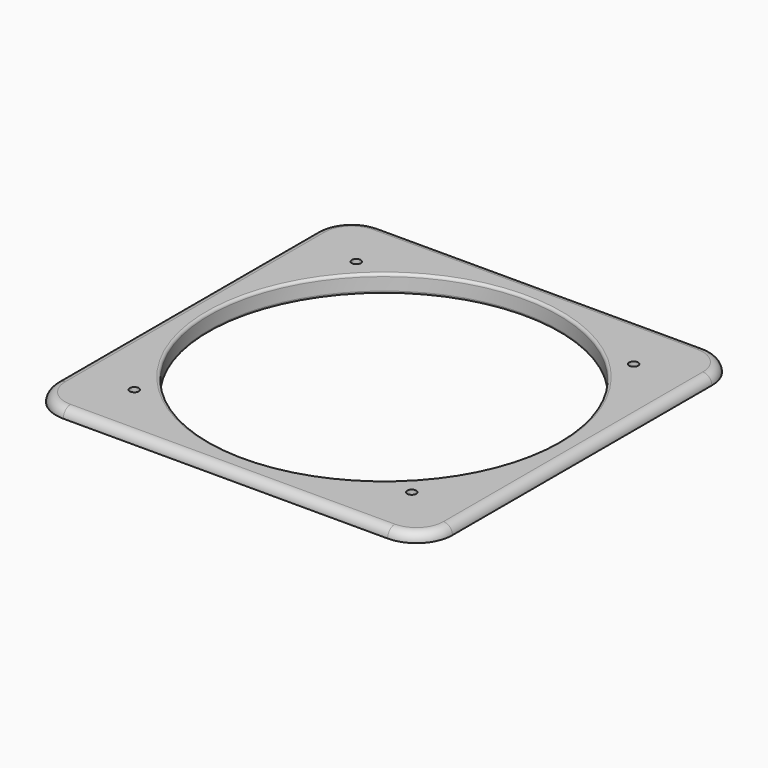
from build123d import *

# Parameters (mm, degrees)
F0_R     = 97
F1_DEPTH = 5
F3_R     = 102
F3_R_2   = 97
F4_DEPTH = 5
F5_R     = 1.5
F6_R     = 4.99999
F2_R     = 2.5
F7_DEPTH = 5


# Not quite as in the source:
# - a fillet or chamfer is up to 0.001 mm smaller than in the source, because OpenCascade refuses the exact size


with BuildPart() as f1:
    # F0 (on Top) → F1 (new body)
    with BuildSketch(Plane.XY):
        with BuildLine():
            Line((-90, -110), (90, -110))
            ThreePointArc((90, -110), (104.1421356237, -104.1421356237), (110, -90))
            Line((110, -90), (110, 90))
            ThreePointArc((110, 90), (104.1421356237, 104.1421356237), (90, 110))
            Line((90, 110), (-90, 110))
            ThreePointArc((-90, 110), (-104.1421356237, 104.1421356237), (-110, 90))
            Line((-110, 90), (-110, -90))
            ThreePointArc((-110, -90), (-104.1421356237, -104.1421356237), (-90, -110))
        make_face()
        Circle(F0_R, mode=Mode.SUBTRACT)
    extrude(amount=F1_DEPTH)

    # F3 (on face) → F4 (join)
    with BuildSketch(Plane(origin=(0, 0, 0), x_dir=(1, 0, 0), z_dir=(0, 0, -1))):
        Circle(F3_R)
        Circle(F3_R_2, mode=Mode.SUBTRACT)
    extrude(amount=F4_DEPTH)

    # F5
    f5_edges = [f1.edges().sort_by_distance(p)[0] for p in [
        (-97, 0, -5),
        (-102, 0, -5),
        (-97, 0, 5),
    ]]
    fillet(f5_edges, radius=F5_R)

    # F6 (radius 5 in the source; OpenCascade refuses exactly that, so slightly less here)
    f6_edges = [f1.edges().sort_by_distance(p)[0] for p in [
        (-98.5, 0, 5),
        (0, -110, 5),
        (104.142136, -104.142136, 5),
        (110, 0, 5),
        (104.142136, 104.142136, 5),
        (0, 110, 5),
        (-104.142136, 104.142136, 5),
        (-110, 0, 5),
        (-104.142136, -104.142136, 5),
    ]]
    fillet(f6_edges, radius=F6_R)

    # F2 (on face) → F7 (cut, through all)
    with BuildSketch(Plane(origin=(0, 0, 0), x_dir=(1, 0, 0), z_dir=(0, 0, -1))):
        with Locations((-77, 77)):
            Circle(F2_R)
        with Locations((77, 77)):
            Circle(F2_R)
        with Locations((77, -77)):
            Circle(F2_R)
        with Locations((-77, -77)):
            Circle(F2_R)
    extrude(amount=-F7_DEPTH, mode=Mode.SUBTRACT)


solid = f1.part
